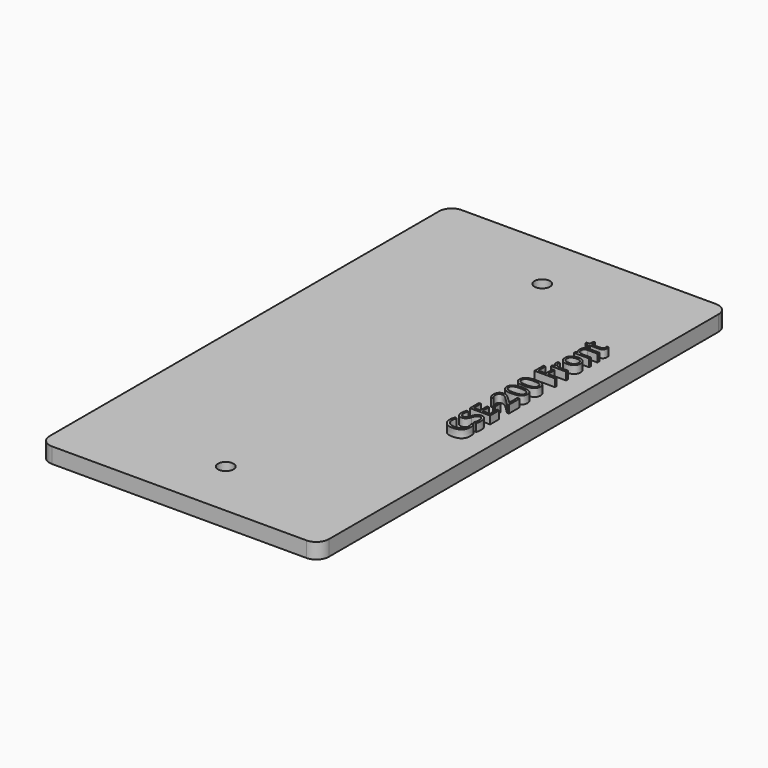
from build123d import *

# Parameters (mm, degrees)
F0_W         = 114.3
F0_H         = 209.55
F0_R         = 3.175
F1_DEPTH     = 6.35
F2_R         = 5.08
F3_TEXT_SIZE = 11.5951401603
F4_DEPTH     = 3.175


# Not quite as in the source:
# - Text() gives the source's letters only with a copy of the font that has no kerning and outlines rounded to 1/6400 em; it was checked with that copy


with BuildPart() as f1:
    # F0 (on Top) → F1 (new body)
    with BuildSketch(Plane.XY):
        with Locations((0, 16.7900487542)):
            Rectangle(F0_W, F0_H)
        with Locations((0, -64.1724512458)):
            Circle(F0_R, mode=Mode.SUBTRACT)
        with Locations((0, 97.7525487542)):
            Circle(F0_R, mode=Mode.SUBTRACT)
    extrude(amount=F1_DEPTH)

    # F2
    f2_edges = [f1.edges().sort_by_distance(p)[0] for p in [
        (57.15, 121.565049, 3.175),
        (-57.15, 121.565049, 3.175),
        (-57.15, -87.984951, 3.175),
        (57.15, -87.984951, 3.175),
    ]]
    fillet(f2_edges, radius=F2_R)

    # F3 (on face) → F4 (join)
    with BuildSketch(Plane.XY.offset(6.35)):
        with Locations(Location((47.7850995958, -3.4609474764), (0, 0, 90))):
            Text('CSE-200 Front', F3_TEXT_SIZE, font='Open Sans', text_align=(TextAlign.LEFT, TextAlign.BOTTOM))
    extrude(amount=F4_DEPTH)


solid = f1.part
